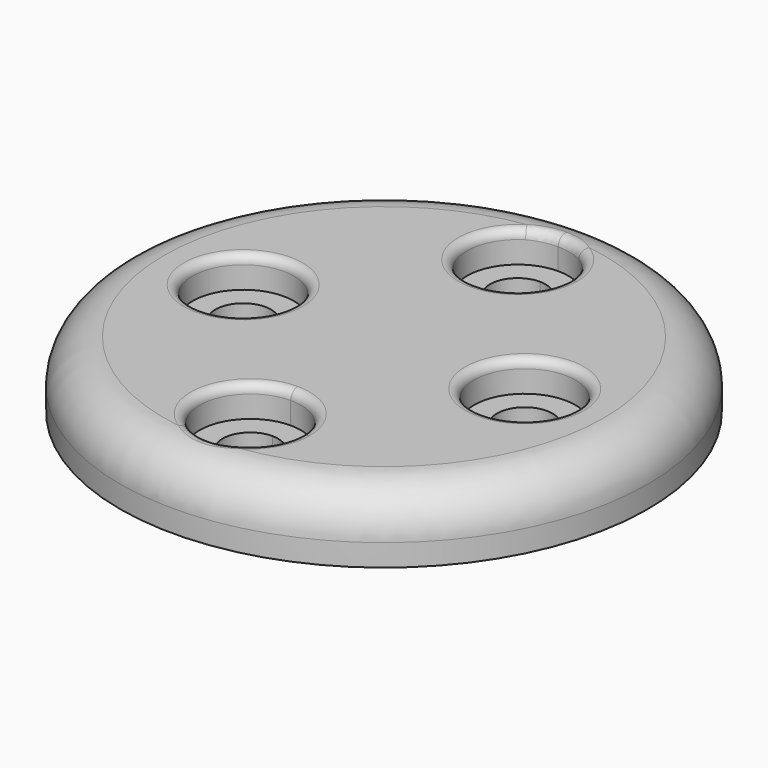
from build123d import *

# Parameters (mm, degrees)
F1_DEPTH = 2
F2_DEPTH = 3.75
F4_R     = 0.5


# Not quite as in the source:
# - a fillet or chamfer that OpenCascade refuses, or shapes differently, is made with other operations: its cross-section is extruded or revolved along the edge and cut away or added


with BuildPart() as f1:
    # F0 (on Top) → F1 (new body)
    with BuildSketch(Plane.XY):
        with BuildLine():
            Line((10.875, 0), (15, 0))
            ThreePointArc((15, 0), (10.6066017178, 10.6066017178), (0, 15))
            Line((0, 15), (0, 12.375))
            ThreePointArc((0, 12.375), (2.0329319959, 11.5329319959), (2.875, 9.5))
            ThreePointArc((2.875, 9.5), (2.0329319959, 7.4670680041), (0, 6.625))
            Line((0, 6.625), (0, 0))
            Line((0, 0), (5.125, 0))
            ThreePointArc((5.125, 0), (8, 2.875), (10.875, 0))
        make_face()
        with BuildLine():
            ThreePointArc((0, -15), (10.6066017178, -10.6066017178), (15, 0))
            Line((15, 0), (10.875, 0))
            ThreePointArc((10.875, 0), (8, -2.875), (5.125, 0))
            Line((5.125, 0), (0, 0))
            Line((0, 0), (0, -6.625))
            ThreePointArc((0, -6.625), (2.0329319959, -7.4670680041), (2.875, -9.5))
            ThreePointArc((2.875, -9.5), (2.0329319959, -11.5329319959), (0, -12.375))
            Line((0, -12.375), (0, -15))
        make_face()
        with BuildLine():
            Line((0, 12.375), (0, 15))
            ThreePointArc((0, 15), (-10.6066017178, 10.6066017178), (-15, 0))
            Line((-15, 0), (-10.875, 0))
            ThreePointArc((-10.875, 0), (-8, 2.875), (-5.125, 0))
            Line((-5.125, 0), (0, 0))
            Line((0, 0), (0, 6.625))
            ThreePointArc((0, 6.625), (-2.875, 9.5), (0, 12.375))
        make_face()
        with BuildLine():
            ThreePointArc((-15, 0), (-10.6066017178, -10.6066017178), (0, -15))
            Line((0, -15), (0, -12.375))
            ThreePointArc((0, -12.375), (-2.875, -9.5), (0, -6.625))
            Line((0, -6.625), (0, 0))
            Line((0, 0), (-5.125, 0))
            ThreePointArc((-5.125, 0), (-8, -2.875), (-10.875, 0))
            Line((-10.875, 0), (-15, 0))
        make_face()
        with BuildLine():
            ThreePointArc((-5.125, 0), (-8, 2.875), (-10.875, 0))
            Line((-10.875, 0), (-9.575, 0))
            ThreePointArc((-9.575, 0), (-8, 1.575), (-6.425, 0))
            Line((-6.425, 0), (-5.125, 0))
        make_face()
        with BuildLine():
            Line((-9.575, 0), (-10.875, 0))
            ThreePointArc((-10.875, 0), (-8, -2.875), (-5.125, 0))
            Line((-5.125, 0), (-6.425, 0))
            ThreePointArc((-6.425, 0), (-8, -1.575), (-9.575, 0))
        make_face()
        with BuildLine():
            ThreePointArc((0, -6.625), (-2.875, -9.5), (0, -12.375))
            Line((0, -12.375), (0, -11.075))
            ThreePointArc((0, -11.075), (-1.575, -9.5), (0, -7.925))
            Line((0, -7.925), (0, -6.625))
        make_face()
        with BuildLine():
            Line((0, -11.075), (0, -12.375))
            ThreePointArc((0, -12.375), (2.0329319959, -11.5329319959), (2.875, -9.5))
            ThreePointArc((2.875, -9.5), (2.0329319959, -7.4670680041), (0, -6.625))
            Line((0, -6.625), (0, -7.925))
            ThreePointArc((0, -7.925), (1.1136931804, -8.3863068196), (1.575, -9.5))
            ThreePointArc((1.575, -9.5), (1.1136931804, -10.6136931804), (0, -11.075))
        make_face()
        with BuildLine():
            ThreePointArc((5.125, 0), (8, -2.875), (10.875, 0))
            Line((10.875, 0), (9.575, 0))
            ThreePointArc((9.575, 0), (8, -1.575), (6.425, 0))
            Line((6.425, 0), (5.125, 0))
        make_face()
        with BuildLine():
            Line((9.575, 0), (10.875, 0))
            ThreePointArc((10.875, 0), (8, 2.875), (5.125, 0))
            Line((5.125, 0), (6.425, 0))
            ThreePointArc((6.425, 0), (8, 1.575), (9.575, 0))
        make_face()
        with BuildLine():
            ThreePointArc((2.875, 9.5), (2.0329319959, 11.5329319959), (0, 12.375))
            Line((0, 12.375), (0, 11.075))
            ThreePointArc((0, 11.075), (1.1136931804, 10.6136931804), (1.575, 9.5))
            ThreePointArc((1.575, 9.5), (1.1136931804, 8.3863068196), (0, 7.925))
            Line((0, 7.925), (0, 6.625))
            ThreePointArc((0, 6.625), (2.0329319959, 7.4670680041), (2.875, 9.5))
        make_face()
        with BuildLine():
            Line((0, 11.075), (0, 12.375))
            ThreePointArc((0, 12.375), (-2.875, 9.5), (0, 6.625))
            Line((0, 6.625), (0, 7.925))
            ThreePointArc((0, 7.925), (-1.575, 9.5), (0, 11.075))
        make_face()
    extrude(amount=F1_DEPTH)

    # F0 (on Top) → F2 (join)
    with BuildSketch(Plane.XY):
        with BuildLine():
            Line((0, 12.375), (0, 15))
            ThreePointArc((0, 15), (-10.6066017178, 10.6066017178), (-15, 0))
            Line((-15, 0), (-10.875, 0))
            ThreePointArc((-10.875, 0), (-8, 2.875), (-5.125, 0))
            Line((-5.125, 0), (0, 0))
            Line((0, 0), (0, 6.625))
            ThreePointArc((0, 6.625), (-2.875, 9.5), (0, 12.375))
        make_face()
        with BuildLine():
            ThreePointArc((-15, 0), (-10.6066017178, -10.6066017178), (0, -15))
            Line((0, -15), (0, -12.375))
            ThreePointArc((0, -12.375), (-2.875, -9.5), (0, -6.625))
            Line((0, -6.625), (0, 0))
            Line((0, 0), (-5.125, 0))
            ThreePointArc((-5.125, 0), (-8, -2.875), (-10.875, 0))
            Line((-10.875, 0), (-15, 0))
        make_face()
        with BuildLine():
            ThreePointArc((0, -15), (10.6066017178, -10.6066017178), (15, 0))
            Line((15, 0), (10.875, 0))
            ThreePointArc((10.875, 0), (8, -2.875), (5.125, 0))
            Line((5.125, 0), (0, 0))
            Line((0, 0), (0, -6.625))
            ThreePointArc((0, -6.625), (2.0329319959, -7.4670680041), (2.875, -9.5))
            ThreePointArc((2.875, -9.5), (2.0329319959, -11.5329319959), (0, -12.375))
            Line((0, -12.375), (0, -15))
        make_face()
        with BuildLine():
            Line((10.875, 0), (15, 0))
            ThreePointArc((15, 0), (10.6066017178, 10.6066017178), (0, 15))
            Line((0, 15), (0, 12.375))
            ThreePointArc((0, 12.375), (2.0329319959, 11.5329319959), (2.875, 9.5))
            ThreePointArc((2.875, 9.5), (2.0329319959, 7.4670680041), (0, 6.625))
            Line((0, 6.625), (0, 0))
            Line((0, 0), (5.125, 0))
            ThreePointArc((5.125, 0), (8, 2.875), (10.875, 0))
        make_face()
    extrude(amount=F2_DEPTH)

    # F3: fillet of radius 2.5 on 1 edges, made by hand

    # F3_s1 → F3_t2 (revolve, cut)
    with BuildSketch(Plane.XZ):
        with BuildLine():
            ThreePointArc((15, 1.25), (14.267766953, 3.017766953), (12.5, 3.75))
            Line((12.5, 3.75), (15, 3.75))
            Line((15, 3.75), (15, 1.25))
        make_face()
    revolve(axis=Axis((0, 0, 3.75), (0, 0, 1)), mode=Mode.SUBTRACT)

    # F4
    f4_edges = [f1.edges().sort_by_distance(p)[0] for p in [
        (0, 6.625, 3.75),
        (-10.875, 0, 3.75),
        (0, -12.375, 3.75),
        (10.875, 0, 3.75),
    ]]
    fillet(f4_edges, radius=F4_R)


solid = f1.part
